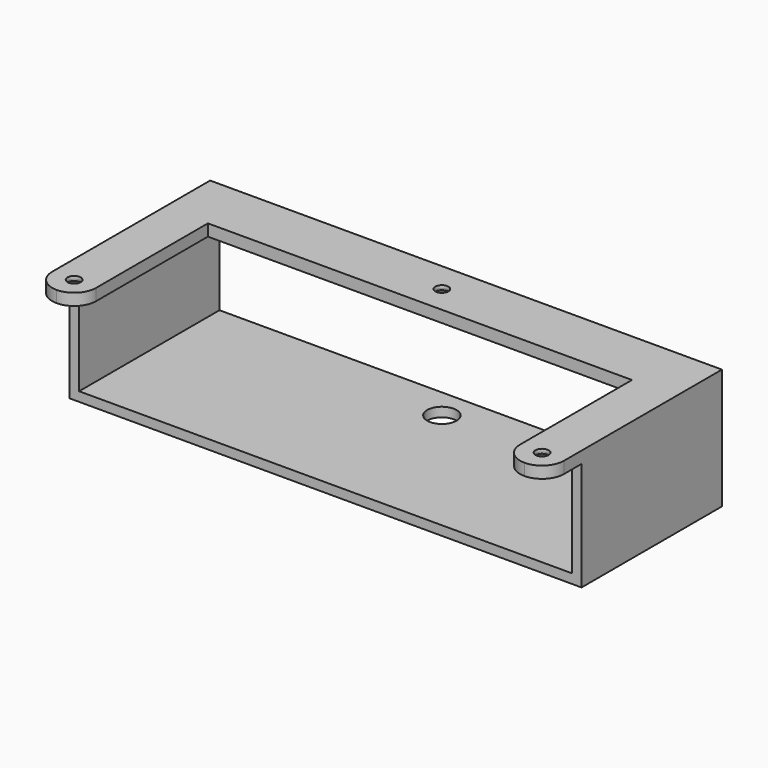
from build123d import *

# Parameters (mm, degrees)
F0_W      = 3.2
F0_H      = 60
F0_W_2    = 168.6
F1_DEPTH  = 3
F2_DEPTH  = 37.2
F3_W      = 60
F3_H      = 3.2
F4_DEPTH  = 168.6
F5_W      = 15
F5_H      = 3
F6_DEPTH  = 15
F7_W      = 15
F7_H      = 3
F8_DEPTH  = 15
F9_R      = 2.25
F10_DEPTH = 25
F11_DEPTH = 1
F12_SIZE  = 2.5
F13_W     = 35.8230434358
F13_H     = 13.5607076809
F14_DEPTH = 175.001
F15_R     = 5
F16_DEPTH = 25
F17_R     = 7.49999
F18_DEPTH = 40.3


# Not quite as in the source:
# - a fillet or chamfer is up to 0.001 mm smaller than in the source, because OpenCascade refuses the exact size


with BuildPart() as f1:
    # F0 (on Top) → F1 (new body)
    with BuildSketch(Plane.XY):
        with Locations((1.6, -30)):
            Rectangle(F0_W, F0_H)
        with Locations((87.5, -30)):
            Rectangle(F0_W_2, F0_H)
        with Locations((173.4, -30)):
            Rectangle(F0_W, F0_H)
    extrude(amount=F1_DEPTH)

    # F0 (on Top) → F2 (join)
    with BuildSketch(Plane.XY):
        with Locations((1.6, -30)):
            Rectangle(F0_W, F0_H)
        with Locations((173.4, -30)):
            Rectangle(F0_W, F0_H)
    extrude(amount=-F2_DEPTH)

    # F3 (on face) → F4 (join, through all)
    with BuildSketch(Plane(origin=(171.8, 0, 0), x_dir=(0, -1, 0), z_dir=(-1, 0, 0))):
        with Locations((30, -35.6)):
            Rectangle(F3_W, F3_H)
    extrude(amount=F4_DEPTH)

    # F5 (on face) → F6 (join)
    with BuildSketch(Plane.XZ.offset(60)):
        with Locations((7.5, 1.5)):
            Rectangle(F5_W, F5_H)
        with Locations((167.5, 1.5)):
            Rectangle(F5_W, F5_H)
    extrude(amount=F6_DEPTH)

    # F7 (on face) → F8 (join)
    with BuildSketch(Plane(origin=(0, 0, 0), x_dir=(-1, 0, 0), z_dir=(0, 1, 0))):
        with Locations((-167.5, 1.5)):
            Rectangle(F7_W, F7_H)
        with Locations((-7.5, 1.5)):
            Rectangle(F7_W, F7_H)
    extrude(amount=F8_DEPTH)

    # F9 (on face) → F10 (cut)
    with BuildSketch(Plane.XY.offset(3)):
        with Locations((167.5, 7.5)):
            Circle(F9_R)
        with Locations((167.5, -67.5)):
            Circle(F9_R)
        with Locations((7.5, -67.5)):
            Circle(F9_R)
        with Locations((87.5, -10.3430738673)):
            Circle(F9_R)
    extrude(amount=-F10_DEPTH, mode=Mode.SUBTRACT)

    # F11 (add): a face of the model
    f11_faces = [f1.faces().sort_by_distance(p)[0] for p in [
        (87.3877644613, -29.9749671624, 3),
    ]]
    extrude(f11_faces, amount=F11_DEPTH)

    # F12
    f12_edges = [f1.edges().sort_by_distance(p)[0] for p in [
        (165.25, -67.5, 0),
        (165.25, 7.5, 0),
        (85.25, -10.343074, 0),
        (5.25, -67.5, 0),
    ]]
    chamfer(f12_edges, length=F12_SIZE)

    # F13 (on face) → F14 (cut, through all)
    with BuildSketch(Plane(origin=(0, 0, 0), x_dir=(0, -1, 0), z_dir=(-1, 0, 0))):
        with Locations((-17.9115217179, 6.7803538404)):
            Rectangle(F13_W, F13_H)
    extrude(amount=-F14_DEPTH, mode=Mode.SUBTRACT)

    # F15 (on face) → F16 (cut)
    with BuildSketch(Plane.XY.offset(-34)):
        with Locations((87.5478237867, -10.3831542656)):
            Circle(F15_R)
    extrude(amount=-F16_DEPTH, mode=Mode.SUBTRACT)

    # F17 (radius 7.5 in the source; OpenCascade refuses exactly that, so slightly less here)
    f17_edges = [f1.edges().sort_by_distance(p)[0] for p in [
        (15, -75, 2),
        (0, -75, 2),
        (160, -75, 2),
        (175, -75, 2),
    ]]
    fillet(f17_edges, radius=F17_R)

    # F18 (cut): a face of the model
    f18_faces = [f1.faces().sort_by_distance(p)[0] for p in [
        (87.5, -60, 2),
    ]]
    extrude(f18_faces, amount=-F18_DEPTH, mode=Mode.SUBTRACT)


solid = f1.part
